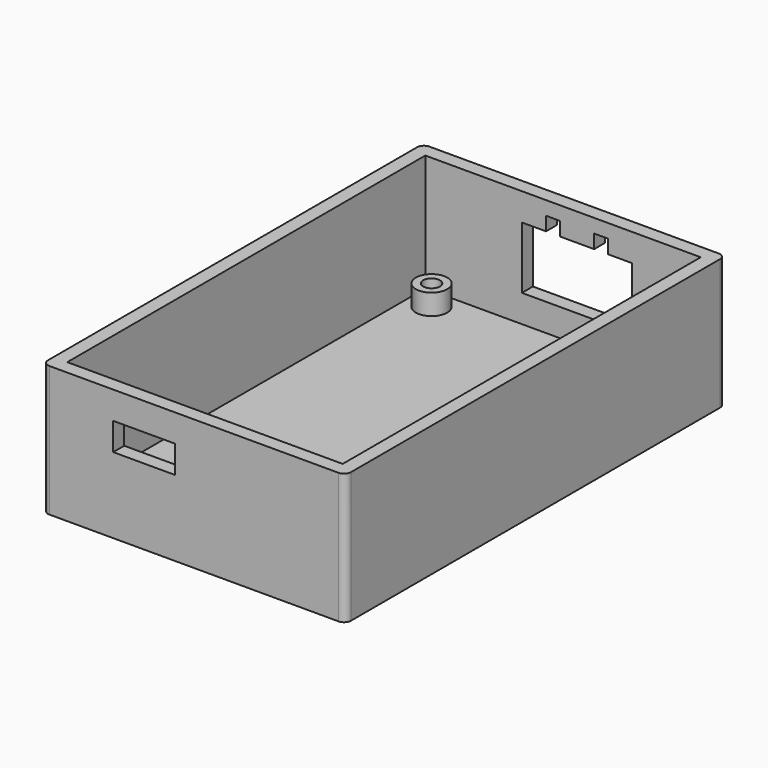
from build123d import *

# Parameters (mm, degrees)
F0_W     = 40
F0_H     = 65
F0_R     = 2.2837988166
F0_R_2   = 1.2192556023
F1_DEPTH = 2
F2_DEPTH = 19
F3_DEPTH = 5
F5_DEPTH = 5
F6_W     = 9
F6_H     = 4
F7_DEPTH = 5


with BuildPart() as f1:
    # F0 (on Top) → F1 (new body)
    with BuildSketch(Plane.XY):
        with BuildLine():
            ThreePointArc((22, 33.5), (21.7071067812, 34.2071067812), (21, 34.5))
            Line((21, 34.5), (-21, 34.5))
            ThreePointArc((-21, 34.5), (-21.7071067812, 34.2071067812), (-22, 33.5))
            Line((-22, 33.5), (-22, -33.5))
            ThreePointArc((-22, -33.5), (-21.7071067812, -34.2071067812), (-21, -34.5))
            Line((-21, -34.5), (21, -34.5))
            ThreePointArc((21, -34.5), (21.7071067812, -34.2071067812), (22, -33.5))
            Line((22, -33.5), (22, 33.5))
        make_face()
        Rectangle(F0_W, F0_H, mode=Mode.SUBTRACT)
        Rectangle(F0_W, F0_H)
        with Locations((-16.6275631636, -29.5829899758)):
            Circle(F0_R, mode=Mode.SUBTRACT)
        with Locations((17.0274368364, -29.5829899758)):
            Circle(F0_R, mode=Mode.SUBTRACT)
        with Locations((-16.6275631636, 29.4170100242)):
            Circle(F0_R, mode=Mode.SUBTRACT)
        with Locations((17.0274368364, 29.4170100242)):
            Circle(F0_R, mode=Mode.SUBTRACT)
        with Locations((17.0274368364, -29.5829899758)):
            Circle(F0_R)
        with Locations((17.0274368364, -29.5829899758)):
            Circle(F0_R_2, mode=Mode.SUBTRACT)
        with Locations((-16.6275631636, -29.5829899758)):
            Circle(F0_R)
        with Locations((-16.6275631636, -29.5829899758)):
            Circle(F0_R_2, mode=Mode.SUBTRACT)
        with Locations((17.0274368364, 29.4170100242)):
            Circle(F0_R)
        with Locations((17.0274368364, 29.4170100242)):
            Circle(F0_R_2, mode=Mode.SUBTRACT)
        with Locations((-16.6275631636, 29.4170100242)):
            Circle(F0_R)
        with Locations((-16.6275631636, 29.4170100242)):
            Circle(F0_R_2, mode=Mode.SUBTRACT)
        with Locations((-16.6275631636, -29.5829899758)):
            Circle(F0_R_2)
        with Locations((17.0274368364, -29.5829899758)):
            Circle(F0_R_2)
        with Locations((17.0274368364, 29.4170100242)):
            Circle(F0_R_2)
        with Locations((-16.6275631636, 29.4170100242)):
            Circle(F0_R_2)
    extrude(amount=F1_DEPTH)

    # F0 (on Top) → F2 (join)
    with BuildSketch(Plane.XY):
        with BuildLine():
            ThreePointArc((22, 33.5), (21.7071067812, 34.2071067812), (21, 34.5))
            Line((21, 34.5), (-21, 34.5))
            ThreePointArc((-21, 34.5), (-21.7071067812, 34.2071067812), (-22, 33.5))
            Line((-22, 33.5), (-22, -33.5))
            ThreePointArc((-22, -33.5), (-21.7071067812, -34.2071067812), (-21, -34.5))
            Line((-21, -34.5), (21, -34.5))
            ThreePointArc((21, -34.5), (21.7071067812, -34.2071067812), (22, -33.5))
            Line((22, -33.5), (22, 33.5))
        make_face()
        Rectangle(F0_W, F0_H, mode=Mode.SUBTRACT)
    extrude(amount=F2_DEPTH)

    # F0 (on Top) → F3 (join)
    with BuildSketch(Plane.XY):
        with Locations((-16.6275631636, 29.4170100242)):
            Circle(F0_R)
        with Locations((-16.6275631636, 29.4170100242)):
            Circle(F0_R_2, mode=Mode.SUBTRACT)
        with Locations((17.0274368364, 29.4170100242)):
            Circle(F0_R)
        with Locations((17.0274368364, 29.4170100242)):
            Circle(F0_R_2, mode=Mode.SUBTRACT)
        with Locations((-16.6275631636, -29.5829899758)):
            Circle(F0_R)
        with Locations((-16.6275631636, -29.5829899758)):
            Circle(F0_R_2, mode=Mode.SUBTRACT)
        with Locations((17.0274368364, -29.5829899758)):
            Circle(F0_R)
        with Locations((17.0274368364, -29.5829899758)):
            Circle(F0_R_2, mode=Mode.SUBTRACT)
    extrude(amount=F3_DEPTH)

    # F4 (on face) → F5 (cut)
    with BuildSketch(Plane(origin=(0, 34.5, 0), x_dir=(-1, 0, 0), z_dir=(0, 1, 0))):
        Polygon((-10.027, 6), (5.973, 6), (5.973, 15), (2.473, 15), (2.473, 17), (0.473, 17), (0.473, 15), (-4.527, 15), (-4.527, 17), (-6.527, 17), (-6.527, 15), (-10.027, 15), align=None)
    extrude(amount=-F5_DEPTH, mode=Mode.SUBTRACT)

    # F6 (on face) → F7 (cut)
    with BuildSketch(Plane.XZ.offset(34.5)):
        with Locations((-7.2275631636, 13)):
            Rectangle(F6_W, F6_H)
    extrude(amount=-F7_DEPTH, mode=Mode.SUBTRACT)


solid = f1.part
